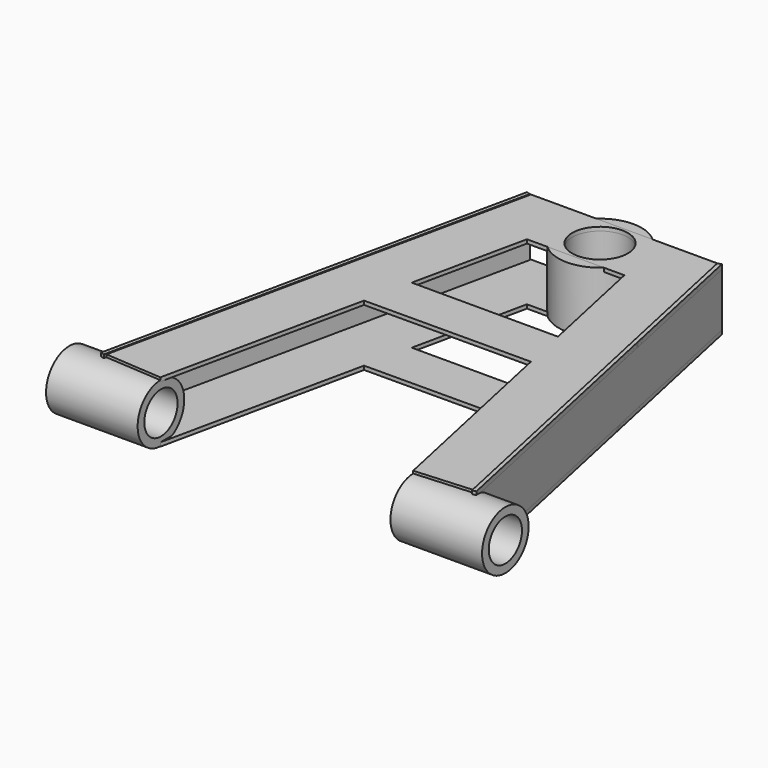
from build123d import *

# Parameters (mm, degrees)
F1_DEPTH  = 3.175
F3_DEPTH  = 3.175
F7_W      = 357.0883721113
F7_H      = 51.4995157719
F8_DEPTH  = 3.175
F10_R     = 24.2355196554
F10_R_2   = 17.2845850153
F19_DEPTH = 76.2
F20_R     = 34.5625940256
F20_R_2   = 23.1276455752
F12_DEPTH = 50.8
F21_DEPTH = 63.5


# Not quite as in the source:
# - a feature of the source that left no trace in its solid (it failed there, or was rolled back) is left out
# - a feature names something its author has since deleted; it is built from what else it names


with BuildPart() as f1:
    # F0 (on face) → F1 (new body)
    with BuildSketch(Plane.XY):
        Polygon((0, 254.7029479625), (-81.0354214167, 254.7029479625), (-155.8285728535, -92.9424813159), (-105.1563591477, -96.5434198266), (-40.5177107084, 203.9029479625), (0, 203.9029479625), align=None)
    extrude(amount=F1_DEPTH)

    # F2: F1 across plane


with BuildPart() as f1_1:
    add(f1.part)
    add(f1.part.mirror(Plane.YZ))

    # F17 (on Top) → F3 (join)
    with BuildSketch(Plane.XY):
        Polygon((64.138263464, 109.4782650471), (-71.3108032942, 109.4782650471), (-85.4815393686, 70.3290700912), (86.3957703114, 71.0801482201), align=None)
    extrude(amount=F3_DEPTH)


with BuildPart() as f5_1:
    # F5: instance of F1
    add(f1_1.part.mirror(Plane.XY.offset(25.4)))


with BuildPart() as f8:
    # F7 (on 3pt) → F8 (new body)
    with BuildSketch(Plane(origin=(-129.823703286, 27.9305380776, 0), x_dir=(0.2103294472, 0.977630566, 0), z_dir=(0.977630566, -0.2103294472, 0))):
        with Locations((53.176112473, 25.7497578859)):
            Rectangle(F7_W, F7_H)
    extrude(amount=F8_DEPTH)


with BuildPart() as f18_1:
    # F18: instance of F8
    add(f8.part.mirror(Plane.YZ))


with BuildPart() as f19:
    # F10 (on plane+point) → F19 (new body)
    with BuildSketch(Plane.YZ.offset(105.1563591477)):
        with Locations((-95.8959981799, 24.5158076286)):
            Circle(F10_R)
        with Locations((-95.8959981799, 24.5158076286)):
            Circle(F10_R_2, mode=Mode.SUBTRACT)
    extrude(amount=F19_DEPTH)


with BuildPart() as f11_1:
    # F11: instance of F19
    add(f19.part.mirror(Plane.YZ))


with BuildPart() as f12:
    # F20 (on Top) → F12 (new body)
    with BuildSketch(Plane.XY):
        with Locations((0, 229.2520552874)):
            Circle(F20_R)
        with Locations((0, 229.2520552874)):
            Circle(F20_R_2, mode=Mode.SUBTRACT)
    extrude(amount=F12_DEPTH)


with BuildPart() as f21_tool:
    # F20 (on Top) → F21 (new body, symmetric)
    with BuildSketch(Plane.XY):
        with Locations((0, 229.2520552874)):
            Circle(F20_R_2)
    extrude(amount=F21_DEPTH, both=True)


with BuildPart() as f1_2:
    add(f1_1.part)

    # F21: cut by f21_tool
    add(f21_tool.part, mode=Mode.SUBTRACT)


with BuildPart() as f5_1_1:
    add(f5_1.part)

    # F21: cut by f21_tool
    add(f21_tool.part, mode=Mode.SUBTRACT)


solid = Compound([f8.part, f18_1.part, f19.part, f11_1.part, f12.part, f1_2.part, f5_1_1.part])
